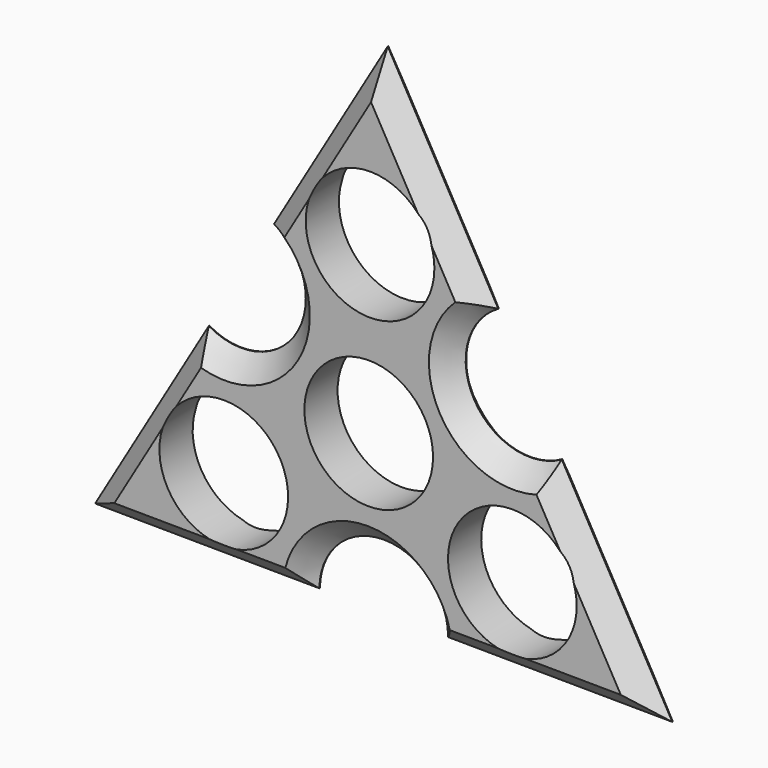
from build123d import *

# Parameters (mm, degrees)
F0_R         = 10.49
F1_DEPTH     = 6.77
F2_T1_DEPTH  = 53.6924086999
F2_T3_DEPTH  = 53.6924086999
F2_T5_DEPTH  = 53.6924086999
F2_T7_DEPTH  = 53.6924086999
F2_T9_DEPTH  = 53.6924086999
F2_T11_DEPTH = 53.6924086999
F2_T14_ANGLE = 273.6993702429
F2_T16_ANGLE = 273.6993702429
F2_T18_ANGLE = 273.6993702439
F2_T20_ANGLE = 273.6993702429
F2_T22_ANGLE = 273.6993702429
F2_T24_ANGLE = 273.6993702429


# Not quite as in the source:
# - a fillet or chamfer that OpenCascade refuses, or shapes differently, is made with other operations: its cross-section is extruded or revolved along the edge and cut away or added


with BuildPart() as f1:
    # F0 (on Front) → F1 (new body)
    with BuildSketch(Plane.XZ):
        with BuildLine():
            Line((18.4621305086, 22.5221560266), (0.4319489998, 54.3327168478))
            Line((0.4319489998, 54.3327168478), (-18.1017140256, 22.8128412157))
            ThreePointArc((-18.1017140256, 22.8128412157), (-14.313385988, 18.9790663983), (-12.9287692735, 13.7702186154))
            ThreePointArc((-12.9287692735, 13.7702186154), (-18.2099214906, 4.66483533), (-28.7358245213, 4.7275960151))
            Line((-28.7358245213, 4.7275960151), (-47.2694875467, -26.792279617))
            Line((-47.2694875467, -26.792279617), (-10.7056430125, -27.0829648061))
            ThreePointArc((-10.7056430125, -27.0829648061), (-0.1742773616, -16.6764412961), (10.2740255001, -27.1663584239))
            ThreePointArc((10.2740255001, -27.1663584239), (10.2739426279, -27.2080555622), (10.2736940127, -27.2497520417))
            Line((10.2736940127, -27.2497520417), (46.8375385469, -27.5404372308))
            Line((46.8375385469, -27.5404372308), (28.8073570381, 4.2701235904))
            ThreePointArc((28.8073570381, 4.2701235904), (14.5087275553, 8.2235265437), (18.4621305086, 22.5221560266))
        make_face()
        with Locations((-23.6347437733, -13.3961398085)):
            Circle(F0_R, mode=Mode.SUBTRACT)
        Circle(F0_R, mode=Mode.SUBTRACT)
        with Locations((23.4187692735, -13.7702186154)):
            Circle(F0_R, mode=Mode.SUBTRACT)
        with Locations((0.2159744999, 27.1663584239)):
            Circle(F0_R, mode=Mode.SUBTRACT)
    extrude(amount=F1_DEPTH)

    # F2: chamfer of 3.33 on 18 edges, made by hand

    # F2_s2 → F2_t1 (cut)
    with BuildSketch(Plane(origin=(-0.9763794466, 0, -1.6605113995), x_dir=(0, 1, 0), z_dir=(-0.5068689464, 0, -0.8620231268))):
        Polygon((-6.77, -23.8372169167), (-3.44, -27.1672169167), (-6.77, -27.1672169167), align=None)
        Polygon((-3.33, -27.1672169167), (0, -23.8372169167), (0, -27.1672169167), align=None)
    extrude(amount=F2_T1_DEPTH, mode=Mode.SUBTRACT)

    # F2_s4 → F2_t3 (cut)
    with BuildSketch(Plane(origin=(28.1913940744, 0, 47.9446094332), x_dir=(0, 1, 0), z_dir=(-0.5068689464, 0, -0.8620231268))):
        Polygon((-6.77, -23.8372169167), (-3.44, -27.1672169167), (-6.77, -27.1672169167), align=None)
        Polygon((-3.33, -27.1672169167), (0, -23.8372169167), (0, -27.1672169167), align=None)
    extrude(amount=F2_T3_DEPTH, mode=Mode.SUBTRACT)

    # F2_s6 → F2_t5 (cut)
    with BuildSketch(Plane(origin=(-0.9498553319, 0, 1.6758251042), x_dir=(0, 1, 0), z_dir=(-0.4930994533, 0, 0.8699729474))):
        Polygon((-6.77, -23.8372169167), (-3.44, -27.1672169167), (-6.77, -27.1672169167), align=None)
        Polygon((-3.33, -27.1672169167), (0, -23.8372169167), (0, -27.1672169167), align=None)
    extrude(amount=F2_T5_DEPTH, mode=Mode.SUBTRACT)

    # F2_s8 → F2_t7 (cut)
    with BuildSketch(Plane(origin=(-55.6169467809, 0, 0.4421587199), x_dir=(0, 1, 0), z_dir=(0.9999683997, 0, -0.0079498206))):
        Polygon((-6.77, -23.8372169167), (-3.44, -27.1672169167), (-6.77, -27.1672169167), align=None)
        Polygon((-3.33, -27.1672169167), (0, -23.8372169167), (0, -27.1672169167), align=None)
    extrude(amount=F2_T7_DEPTH, mode=Mode.SUBTRACT)

    # F2_s10 → F2_t9 (cut)
    with BuildSketch(Plane(origin=(1.9262347785, 0, -0.0153137048), x_dir=(0, 1, 0), z_dir=(0.9999683997, 0, -0.0079498206))):
        Polygon((-3.44, -27.1672169167), (-6.77, -23.8372169167), (-6.77, -27.1672169167), align=None)
        Polygon((-3.33, -27.1672169167), (0, -23.8372169167), (0, -27.1672169167), align=None)
    extrude(amount=F2_T9_DEPTH, mode=Mode.SUBTRACT)

    # F2_s12 → F2_t11 (cut)
    with BuildSketch(Plane(origin=(27.4255527065, 0, -48.3867681532), x_dir=(0, 1, 0), z_dir=(-0.4930994533, 0, 0.8699729474))):
        Polygon((-6.77, -23.8372169167), (-3.44, -27.1672169167), (-6.77, -27.1672169167), align=None)
        Polygon((0, -23.8372169167), (-3.33, -27.1672169167), (0, -27.1672169167), align=None)
    extrude(amount=F2_T11_DEPTH, mode=Mode.SUBTRACT)

    # F2_s13 → F2_t14 (revolve, cut)
    with BuildSketch(Plane(origin=(-4.0831164566, 0, 18.1258589444), x_dir=(0, 1, 0), z_dir=(-0.2197579888, 0, 0.97555442))):
        Polygon((-6.77, 33.6401683275), (-3.44, 30.3101683275), (-6.77, 30.3101683275), align=None)
    revolve(axis=Axis((-23.4187692735, -6.77, 13.7702186154), (0, -1, 0)), revolution_arc=F2_T14_ANGLE, mode=Mode.SUBTRACT)

    # F2_s15 → F2_t16 (revolve, cut)
    with BuildSketch(Plane(origin=(4.3707858991, 0, 18.0586498137), x_dir=(0, 1, 0), z_dir=(0.2352406866, 0, 0.9719371479))):
        Polygon((-6.77, -33.6401683275), (-3.44, -30.3101683275), (-6.77, -30.3101683275), align=None)
    revolve(axis=Axis((23.6347437733, -6.77, 13.3961398085), (0, 1, 0)), revolution_arc=F2_T16_ANGLE, mode=Mode.SUBTRACT)

    # F2_s17 → F2_t18 (revolve, cut)
    with BuildSketch(Plane(origin=(-13.6558960829, 0, -12.59901205), x_dir=(0, 1, 0), z_dir=(-0.7349759161, 0, -0.678093211))):
        Polygon((-6.77, 33.6401683276), (-3.44, 30.3101683277), (-6.77, 30.3101683276), align=None)
    revolve(axis=Axis((-0.2159744998, -6.77, -27.1663584239), (0, -1, 0)), revolution_arc=F2_T18_ANGLE, mode=Mode.SUBTRACT)

    # F2_s19 → F2_t20 (revolve, cut)
    with BuildSketch(Plane(origin=(-17.8246424463, 0, -5.2441132837), x_dir=(0, 1, 0), z_dir=(-0.9593426042, 0, -0.2822441634))):
        Polygon((-3.33, -30.3101683275), (0, -33.6401683275), (0, -30.3101683275), align=None)
    revolve(axis=Axis((-23.4187692735, 0, 13.7702186154), (0, 1, 0)), revolution_arc=F2_T20_ANGLE, mode=Mode.SUBTRACT)

    # F2_s21 → F2_t22 (revolve, cut)
    with BuildSketch(Plane(origin=(13.4538565472, 0, -12.81453653), x_dir=(0, 1, 0), z_dir=(0.7241019176, 0, -0.6896929845))):
        Polygon((0, -33.6401683275), (-3.33, -30.3101683275), (0, -30.3101683275), align=None)
    revolve(axis=Axis((-0.2159744999, 0, -27.1663584239), (0, 1, 0)), revolution_arc=F2_T22_ANGLE, mode=Mode.SUBTRACT)

    # F2_s23 → F2_t24 (revolve, cut)
    with BuildSketch(Plane(origin=(4.3707858991, 0, 18.0586498137), x_dir=(0, 1, 0), z_dir=(0.2352406866, 0, 0.9719371479))):
        Polygon((-3.33, -30.3101683275), (0, -33.6401683275), (0, -30.3101683275), align=None)
    revolve(axis=Axis((23.6347437733, 0, 13.3961398085), (0, 1, 0)), revolution_arc=F2_T24_ANGLE, mode=Mode.SUBTRACT)


solid = f1.part
